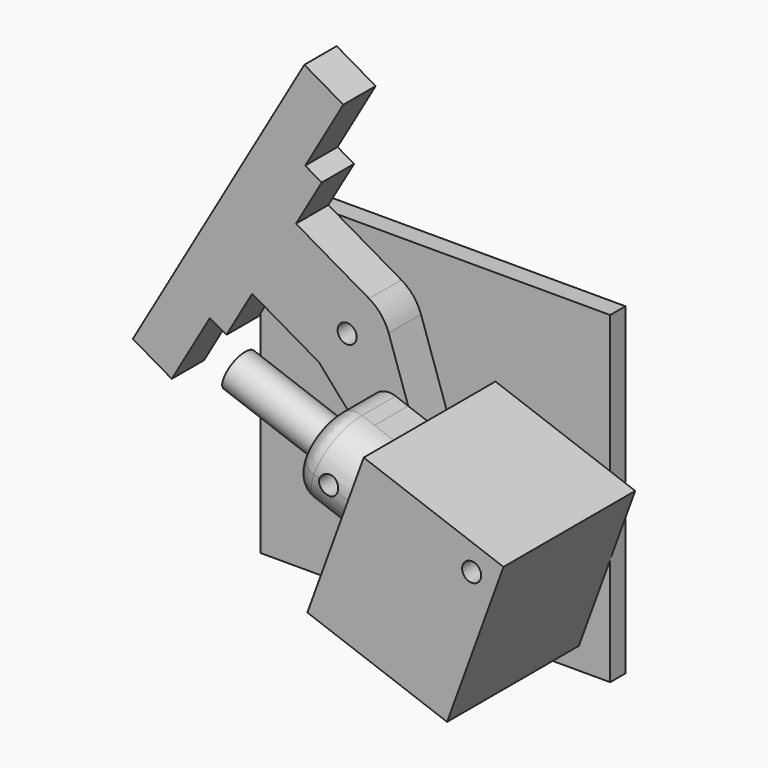
from build123d import *

# Parameters (mm, degrees)
F1_DEPTH    = 10.6
F2_DEPTH    = 43.2
F3_R        = 11
F4_DEPTH    = 2
F5_R        = 5
F6_DEPTH    = 43.4
F8_DEPTH    = 22
F9_T1_DEPTH = 73
F9_T3_DEPTH = 73
F10_W       = 91.6676837951
F10_H       = 84.7782492638
F11_DEPTH   = 5
F12_R       = 2.5
F13_DEPTH   = 74.8
F15_DEPTH   = 10.6
F16_R       = 5


# Not quite as in the source:
# - a fillet or chamfer that OpenCascade refuses, or shapes differently, is made with other operations: its cross-section is extruded or revolved along the edge and cut away or added
# - a feature names something its author has since deleted; it is built from what else it names


with BuildPart() as f1:
    # F0 (on Front) → F1 (new body)
    with BuildSketch(Plane.XZ):
        with BuildLine():
            Line((18.8587860588, -19.9187396285), (10.8963137964, 3.6770022643))
            ThreePointArc((10.8963137964, 3.6770022643), (0.1357629169, 11.4991985995), (-10.806465139, 3.9332316482))
            ThreePointArc((-10.806465139, 3.9332316482), (-11.3009249511, -2.1305152546), (-8.6325342688, -7.5979834231))
            Line((-8.6325342688, -7.5979834231), (-1.2524718249, -15.9829243219))
            ThreePointArc((-1.2524718249, -15.9829243219), (4.0057955945, -16.7858487559), (8.0082155178, -20.289375359))
            Line((8.0082155178, -20.289375359), (10.350768448, -21.1419948978))
            ThreePointArc((10.350768448, -21.1419948978), (13.1341204442, -19.5350258736), (15.2, -21.9970452561))
            ThreePointArc((15.2, -21.9970452561), (15.1620193825, -22.4311657003), (15.049231552, -22.8520956144))
            Line((15.049231552, -22.8520956144), (18.8080020351, -24.2201761877))
            ThreePointArc((18.8080020351, -24.2201761877), (19.1995470345, -22.0737808179), (18.8587860588, -19.9187396285))
        make_face()
        with BuildLine():
            ThreePointArc((2.5, 0), (-0.4341204442, -2.4620193825), (-2.349231552, 0.8550503583))
            ThreePointArc((-2.349231552, 0.8550503583), (0.4341204442, 2.4620193825), (2.5, 0))
        make_face(mode=Mode.SUBTRACT)
        with BuildLine():
            ThreePointArc((8.0082155178, -20.289375359), (4.0057955945, -16.7858487559), (-1.2524718249, -15.9829243219))
            Line((-1.2524718249, -15.9829243219), (-0.0405482356, -17.3598649301))
            Line((-0.0405482356, -17.3598649301), (8.0082155178, -20.289375359))
        make_face()
        with BuildLine():
            ThreePointArc((7.8207415002, -26.2915576257), (8.4967135133, -26.9551076509), (9.2619480899, -27.5133664092))
            ThreePointArc((9.2619480899, -27.5133664092), (9.4402994352, -26.4633656816), (9.5, -25.4))
            ThreePointArc((9.5, -25.4), (9.1194311067, -22.738050284), (8.0082155178, -20.289375359))
            Line((8.0082155178, -20.289375359), (-0.0405482356, -17.3598649301))
            Line((-0.0405482356, -17.3598649301), (7.8207415002, -26.2915576257))
        make_face()
    extrude(amount=F1_DEPTH)

    # F14 (on face) → F15 (join)
    with BuildSketch(Plane.XZ.offset(10.6)):
        with BuildLine():
            Line((-31.664557856, -10.5859724576), (-24.914557856, 1.1053704935))
            Line((-24.914557856, 1.1053704935), (-7.3851056739, -9.0152634426))
            Line((-7.3851056739, -9.0152634426), (-8.6325342688, -7.5979834231))
            ThreePointArc((-8.6325342688, -7.5979834231), (-11.4436081592, -1.137467493), (-9.9592921435, 5.75))
            Line((-9.9592921435, 5.75), (-23.4946848749, 13.564662637))
            Line((-23.4946848749, 13.564662637), (-35.9946848749, -8.0859724576))
            Line((-35.9946848749, -8.0859724576), (-31.664557856, -10.5859724576))
        make_face()
        with BuildLine():
            Line((-17.7446848749, 23.5239547806), (-23.4946848749, 13.564662637))
            Line((-23.4946848749, 13.564662637), (-9.9592921435, 5.75))
            ThreePointArc((-9.9592921435, 5.75), (-2.9764190187, 11.1081470023), (5.75, 9.9592921435))
            Line((5.75, 9.9592921435), (-13.414557856, 21.0239547806))
            Line((-13.414557856, 21.0239547806), (-6.664557856, 32.7152977317))
            Line((-6.664557856, 32.7152977317), (-10.9946848749, 35.2152977317))
            Line((-10.9946848749, 35.2152977317), (-17.7446848749, 23.5239547806))
        make_face()
        Polygon((-41.6238499995, -4.8359724576), (-35.9946848749, -8.0859724576), (-23.4946848749, 13.564662637), (-17.7446848749, 23.5239547806), (-10.9946848749, 35.2152977317), (-16.6238499995, 38.4652977317), align=None)
        Polygon((-45.9946848749, -25.4064805333), (-35.9946848749, -8.0859724576), (-41.6238499995, -4.8359724576), (-16.6238499995, 38.4652977317), (-10.9946848749, 35.2152977317), (-0.9946848749, 52.5358058073), (-11.2137846395, 58.4358058073), (-56.2137846395, -19.5064805333), align=None)
    extrude(amount=-F15_DEPTH)


with BuildPart() as f2:
    # F0 (on Front) → F2 (new body)
    with BuildSketch(Plane.XZ):
        Polygon((30.4242539245, -5.4619062237), (23.0366188286, -25.7592668327), (15.6489837328, -46.0566274417), (52.2969959435, -59.3954130314), (67.0722661351, -18.8006918134), align=None)
    extrude(amount=F2_DEPTH)

    # F3 (on face) → F4 (join)
    with BuildSketch(Plane(origin=(28.6207151126, 0, -10.4170883844), x_dir=(0, -1, 0), z_dir=(-0.9396926208, 0, 0.3420201433))):
        with Locations((21.6, -16.326805286)):
            Circle(F3_R)
    extrude(amount=F4_DEPTH)

    # F5 (on face) → F6 (join)
    with BuildSketch(Plane(origin=(26.7413298711, 0, -9.7330480978), x_dir=(0, -1, 0), z_dir=(-0.9396926208, 0, 0.3420201433))):
        with Locations((21.6, -16.326805286)):
            Circle(F5_R)
    extrude(amount=F6_DEPTH)


with BuildPart() as f8:
    # F7 (on face) → F8 (new body)
    with BuildSketch(Plane.XZ.offset(10.6)):
        with BuildLine():
            ThreePointArc((15.049231552, -22.8520956144), (11.8449496417, -24.3462768081), (10.350768448, -21.1419948978))
            Line((10.350768448, -21.1419948978), (8.0082155178, -20.289375359))
            ThreePointArc((8.0082155178, -20.289375359), (9.3600827685, -23.7755460709), (9.2619480899, -27.5133664092))
            ThreePointArc((9.2619480899, -27.5133664092), (8.4967135133, -26.9551076509), (7.8207415002, -26.2915576257))
            Line((7.8207415002, -26.2915576257), (3.3911070963, -21.2587787078))
            Line((3.3911070963, -21.2587787078), (0.4805448363, -29.2554827948))
            Line((0.4805448363, -29.2554827948), (17.3950120105, -35.4118453747))
            Line((17.3950120105, -35.4118453747), (24.9194551637, -14.7386077174))
            Line((24.9194551637, -14.7386077174), (16.0173460598, -11.4985049814))
            Line((16.0173460598, -11.4985049814), (18.8587860588, -19.9187396285))
            ThreePointArc((18.8587860588, -19.9187396285), (19.1995470345, -22.0737808179), (18.8080020351, -24.2201761877))
            Line((18.8080020351, -24.2201761877), (15.049231552, -22.8520956144))
        make_face()
        with BuildLine():
            ThreePointArc((10.350768448, -21.1419948978), (13.1341204442, -19.5350258736), (15.2, -21.9970452561))
            ThreePointArc((15.2, -21.9970452561), (15.1620193825, -22.4311657003), (15.049231552, -22.8520956144))
            Line((15.049231552, -22.8520956144), (18.8080020351, -24.2201761877))
            ThreePointArc((18.8080020351, -24.2201761877), (19.1995470345, -22.0737808179), (18.8587860588, -19.9187396285))
            Line((18.8587860588, -19.9187396285), (16.0173460598, -11.4985049814))
            Line((16.0173460598, -11.4985049814), (8.0049879895, -8.5822451375))
            Line((8.0049879895, -8.5822451375), (3.3911070963, -21.2587787078))
            Line((3.3911070963, -21.2587787078), (7.8207415002, -26.2915576257))
            ThreePointArc((7.8207415002, -26.2915576257), (8.4967135133, -26.9551076509), (9.2619480899, -27.5133664092))
            ThreePointArc((9.2619480899, -27.5133664092), (9.3600827685, -23.7755460709), (8.0082155178, -20.289375359))
            Line((8.0082155178, -20.289375359), (10.350768448, -21.1419948978))
        make_face()
    extrude(amount=F8_DEPTH)

    # F9: fillet of radius 11 on 2 edges, made by hand

    # F9_s2 → F9_t1 (cut)
    with BuildSketch(Plane(origin=(52.5828769427, 0, -19.1386020392), x_dir=(0, 1, 0), z_dir=(-0.9396926208, 0, 0.3420201433))):
        with BuildLine():
            ThreePointArc((-21.6, 5.326805286), (-29.3781745931, 8.548630693), (-32.6, 16.326805286))
            Line((-32.6, 16.326805286), (-32.6, 5.326805286))
            Line((-32.6, 5.326805286), (-21.6, 5.326805286))
        make_face()
    extrude(amount=F9_T1_DEPTH, mode=Mode.SUBTRACT)

    # F9_s4 → F9_t3 (cut)
    with BuildSketch(Plane(origin=(-16.0146843747, 0, 5.8288684236), x_dir=(0, 1, 0), z_dir=(0.9396926208, 0, -0.3420201433))):
        with BuildLine():
            ThreePointArc((-21.6, -27.326805286), (-29.3781745931, -24.1049798791), (-32.6, -16.326805286))
            Line((-32.6, -16.326805286), (-32.6, -27.326805286))
            Line((-32.6, -27.326805286), (-21.6, -27.326805286))
        make_face()
    extrude(amount=F9_T3_DEPTH, mode=Mode.SUBTRACT)

    # F16
    f16_edges = [f8.edges().sort_by_distance(p)[0] for p in [
        (6.903059, -29.378175, -11.609771),
        (0.480545, -16.1, -29.255483),
        (1.582474, -29.378175, -26.227957),
        (8.004988, -16.1, -8.582245),
    ]]
    fillet(f16_edges, radius=F16_R)


with BuildPart() as f11:
    # F10 (on face) → F11 (new body)
    with BuildSketch(Plane.XZ):
        with Locations((14.6878799424, -22.7255448699)):
            Rectangle(F10_W, F10_H)
        with BuildLine():
            Line((10.8963137964, 3.6770022643), (18.8587860588, -19.9187396285))
            ThreePointArc((18.8587860588, -19.9187396285), (19.1995470345, -22.0737808179), (18.8080020351, -24.2201761877))
            Line((18.8080020351, -24.2201761877), (15.049231552, -22.8520956144))
            ThreePointArc((15.049231552, -22.8520956144), (15.1620193825, -22.4311657003), (15.2, -21.9970452561))
            ThreePointArc((15.2, -21.9970452561), (13.1341204442, -19.5350258736), (10.350768448, -21.1419948978))
            Line((10.350768448, -21.1419948978), (8.0082155178, -20.289375359))
            ThreePointArc((8.0082155178, -20.289375359), (4.0057955945, -16.7858487559), (-1.2524718249, -15.9829243219))
            Line((-1.2524718249, -15.9829243219), (-8.6325342688, -7.5979834231))
            ThreePointArc((-8.6325342688, -7.5979834231), (-11.3009249511, -2.1305152546), (-10.806465139, 3.9332316482))
            ThreePointArc((-10.806465139, 3.9332316482), (0.1357629169, 11.4991985995), (10.8963137964, 3.6770022643))
        make_face(mode=Mode.SUBTRACT)
    extrude(amount=-F11_DEPTH)

    # F0 (on Front) → F11, piece 2 (join)
    with BuildSketch(Plane.XZ):
        with BuildLine():
            Line((18.8587860588, -19.9187396285), (10.8963137964, 3.6770022643))
            ThreePointArc((10.8963137964, 3.6770022643), (0.1357629169, 11.4991985995), (-10.806465139, 3.9332316482))
            ThreePointArc((-10.806465139, 3.9332316482), (-11.3009249511, -2.1305152546), (-8.6325342688, -7.5979834231))
            Line((-8.6325342688, -7.5979834231), (-1.2524718249, -15.9829243219))
            ThreePointArc((-1.2524718249, -15.9829243219), (4.0057955945, -16.7858487559), (8.0082155178, -20.289375359))
            Line((8.0082155178, -20.289375359), (10.350768448, -21.1419948978))
            ThreePointArc((10.350768448, -21.1419948978), (13.1341204442, -19.5350258736), (15.2, -21.9970452561))
            ThreePointArc((15.2, -21.9970452561), (15.1620193825, -22.4311657003), (15.049231552, -22.8520956144))
            Line((15.049231552, -22.8520956144), (18.8080020351, -24.2201761877))
            ThreePointArc((18.8080020351, -24.2201761877), (19.1995470345, -22.0737808179), (18.8587860588, -19.9187396285))
        make_face()
        with BuildLine():
            ThreePointArc((2.5, 0), (-0.4341204442, -2.4620193825), (-2.349231552, 0.8550503583))
            ThreePointArc((-2.349231552, 0.8550503583), (0.4341204442, 2.4620193825), (2.5, 0))
        make_face(mode=Mode.SUBTRACT)
        with BuildLine():
            ThreePointArc((10.350768448, -21.1419948978), (11.8449496417, -24.3462768081), (15.049231552, -22.8520956144))
            Line((15.049231552, -22.8520956144), (10.350768448, -21.1419948978))
        make_face()
        with BuildLine():
            Line((10.350768448, -21.1419948978), (15.049231552, -22.8520956144))
            ThreePointArc((15.049231552, -22.8520956144), (15.1620193825, -22.4311657003), (15.2, -21.9970452561))
            ThreePointArc((15.2, -21.9970452561), (13.1341204442, -19.5350258736), (10.350768448, -21.1419948978))
        make_face()
    extrude(amount=-F11_DEPTH)


with BuildPart() as f13_tool:
    # F12 (on face) → F13 (new body)
    with BuildSketch(Plane.XZ.offset(43.2)):
        with Locations((58.7411331684, -22.6855629169)):
            Circle(F12_R)
    extrude(amount=-F13_DEPTH)


with BuildPart() as f2_1:
    add(f2.part)

    # F13: cut by f13_tool
    add(f13_tool.part, mode=Mode.SUBTRACT)


with BuildPart() as f11_1:
    add(f11.part)

    # F13: cut by f13_tool
    add(f13_tool.part, mode=Mode.SUBTRACT)


solid = Compound([f1.part, f8.part, f2_1.part, f11_1.part])
